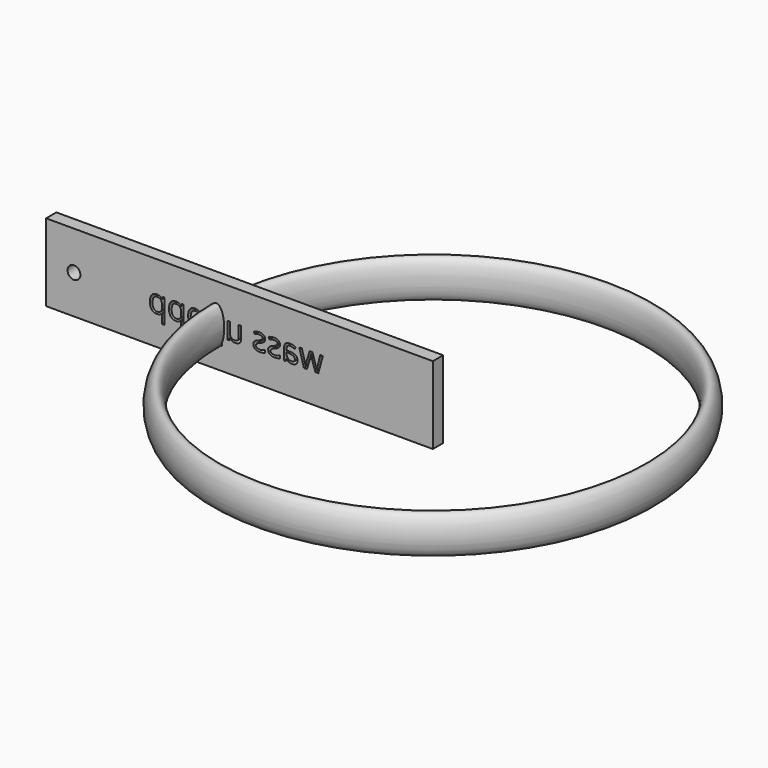
from build123d import *

# Parameters (mm, degrees)
F0_W         = 300
F0_H         = 60
F1_DEPTH     = 10
F2_TEXT_SIZE = 24.1943518631
F3_DEPTH     = 25
F4_R         = 15
F6_R         = 5
F7_DEPTH     = 25


# Not quite as in the source:
# - Text() gives the source's letters only with a copy of the font that has no kerning and outlines rounded to 1/6400 em; it was checked with that copy


with BuildPart() as f1:
    # F0 (on Front) → F1 (new body)
    with BuildSketch(Plane.XZ):
        Rectangle(F0_W, F0_H)
    extrude(amount=-F1_DEPTH)

    # F2 (on face) → F3 (cut)
    with BuildSketch(Plane(origin=(0, 10, 0), x_dir=(-1, 0, 0), z_dir=(0, 1, 0))):
        with Locations((-64.9615898728, -7.1522979997)):
            Text('wass upppp', F2_TEXT_SIZE, font='Open Sans', text_align=(TextAlign.LEFT, TextAlign.BOTTOM))
    extrude(amount=-F3_DEPTH, mode=Mode.SUBTRACT)

    # F4 (on Right) → F5 (revolve)
    with BuildSketch(Plane.YZ):
        with Locations((-75.7319331169, 0)):
            Circle(F4_R)
    revolve(axis=Axis((150, 0, 0), (0, 0, -1)))

    # F6 (on face) → F7 (cut)
    with BuildSketch(Plane(origin=(0, 10, 0), x_dir=(-1, 0, 0), z_dir=(0, 1, 0))):
        with Locations((128.3707022667, 0)):
            Circle(F6_R)
    extrude(amount=-F7_DEPTH, mode=Mode.SUBTRACT)


solid = f1.part
